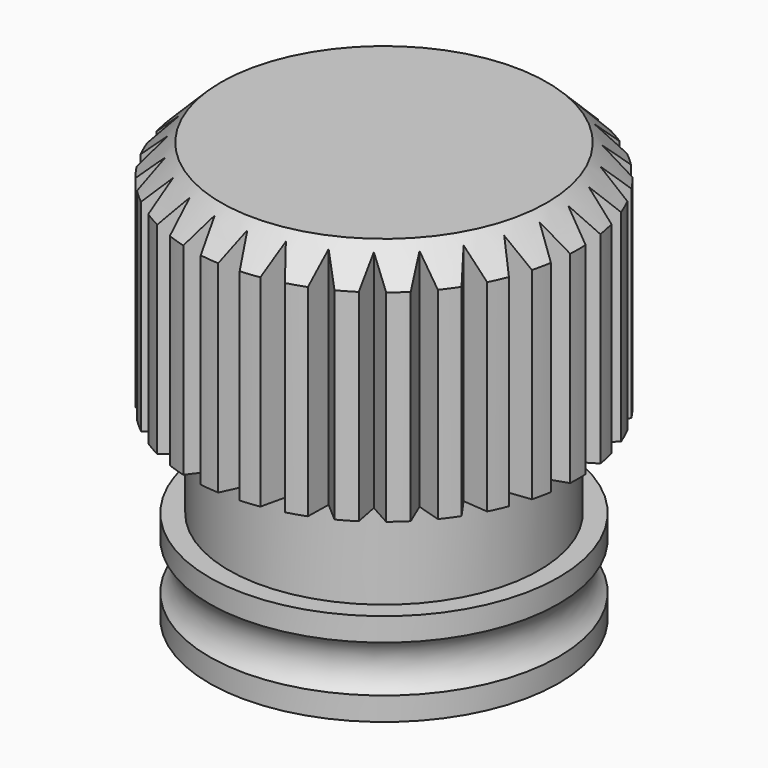
from build123d import *

# Parameters (mm, degrees)
F5_DEPTH        = 15
F5_COPIES_COUNT = 30


# Not quite as in the source:
# - a feature of the source that left no trace in its solid (it failed there, or was rolled back) is left out
# - a pattern or mirror of a feature is missing from the dataset's text; its kind, count and spacing are read off the source's solid


with BuildPart() as f3:
    # F2 (on Front) → F3 (revolve)
    with BuildSketch(Plane.XZ):
        with BuildLine():
            Line((-11.25, 0), (0, 0))
            Line((0, 0), (0, 27))
            Line((0, 27), (-10.5, 27))
            Line((-10.5, 27), (-12.5, 25))
            Line((-12.5, 25), (-12.5, 12))
            Line((-12.5, 12), (-10, 12))
            Line((-10, 12), (-10, 6))
            Line((-10, 6), (-11.25, 6))
            Line((-11.25, 6), (-11.25, 4.5))
            ThreePointArc((-11.25, 4.5), (-10.5728756555, 3), (-11.25, 1.5))
            Line((-11.25, 1.5), (-11.25, 0))
        make_face()
    revolve(axis=Axis((0, 0, 13.5), (0, 0, -1)))

    # F4 (on face) → F5 (cut)
    with BuildSketch(Plane.XY.offset(27)):
        with BuildLine():
            Line((0, 11), (0.6905599091, 12.4809105041))
            ThreePointArc((0.6905599091, 12.4809105041), (0, 12.5), (-0.6905599091, 12.4809105041))
            Line((-0.6905599091, 12.4809105041), (0, 11))
        make_face()
    f5 = extrude(amount=-F5_DEPTH, mode=Mode.SUBTRACT)

    # F5_copies: F5 ×30 about axis
    f5_copies_axis = Axis((0, 0, 0), (0, 0, 1))
    for i in range(1, F5_COPIES_COUNT):
        add(f5.rotate(f5_copies_axis, i * 360 / F5_COPIES_COUNT), mode=Mode.SUBTRACT)


solid = f3.part
